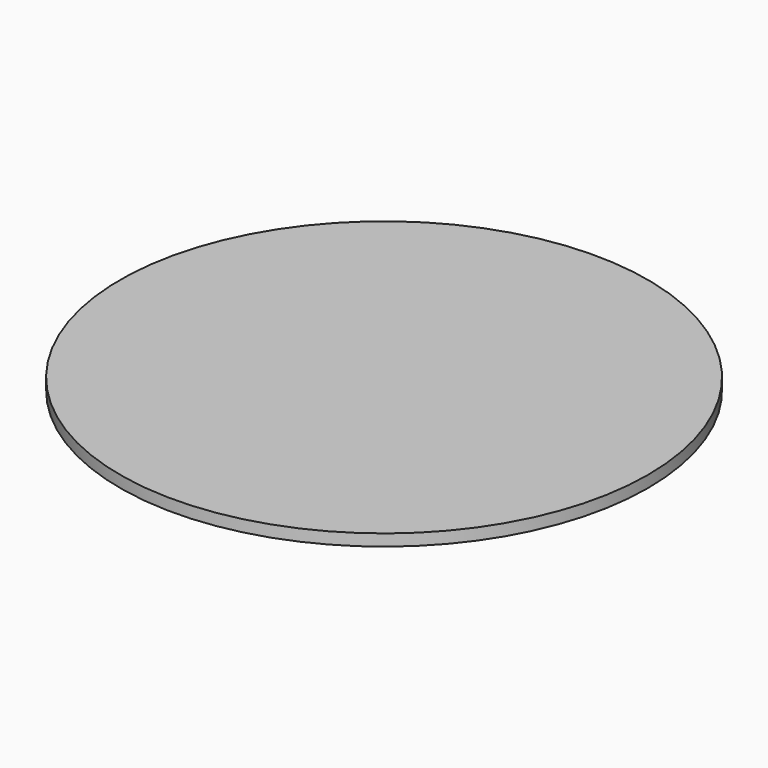
from build123d import *

# Parameters (mm, degrees)
F0_R     = 107.95
F1_DEPTH = 4.7625


# Not quite as in the source:
# - a length typed as a fraction of an inch, garbled in the dataset ("3 / 203.2 mm" for 3/8 in), is restored


with BuildPart() as f1:
    # F0 (on Top) → F1 (new body)
    with BuildSketch(Plane.XY):
        Circle(F0_R)
    extrude(amount=F1_DEPTH)


solid = f1.part
